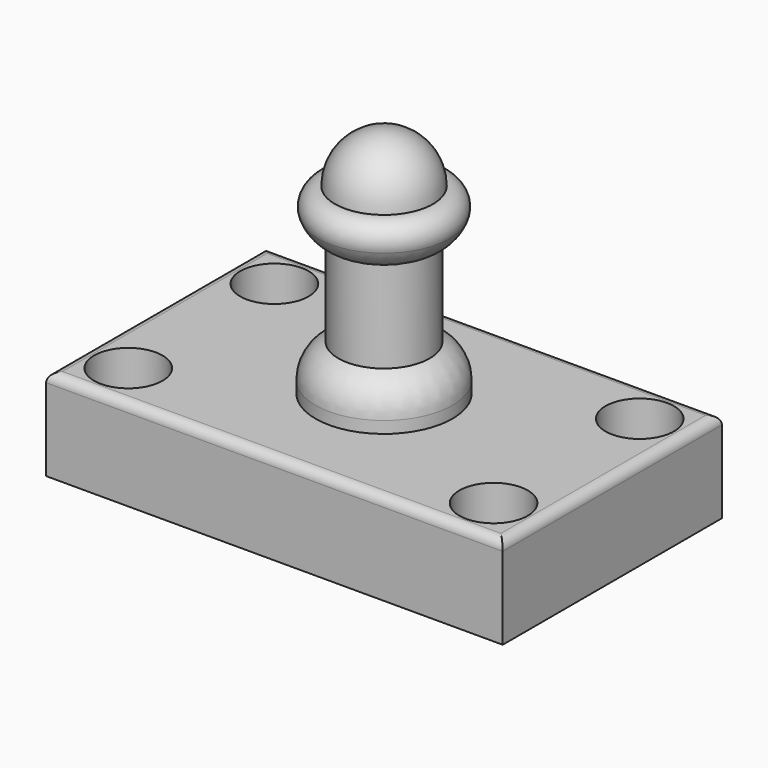
from build123d import *

# Parameters (mm, degrees)
F0_W     = 127
F0_H     = 76.2
F1_DEPTH = 25.4
F3_D     = 19.05
F4_W     = 19.05
F4_H     = 50.8
F6_W     = 12.7
F6_H     = 25.4
F9_R     = 2.54


# Not quite as in the source:
# - a fillet or chamfer that OpenCascade refuses, or shapes differently, is made with other operations: its cross-section is extruded or revolved along the edge and cut away or added


with BuildPart() as f1:
    # F0 (on Top) → F1 (new body)
    with BuildSketch(Plane.XY):
        Rectangle(F0_W, F0_H)
    extrude(amount=F1_DEPTH)

    # F3 (through all)
    with Locations(Plane.XY.offset(25.4)):
        with Locations((-50.8, 25.4), (50.8, 25.4), (-50.8, -25.4), (50.8, -25.4)):
            Hole(F3_D / 2)

    # F4 (on Front) → F5 (revolve)
    with BuildSketch(Plane.XZ):
        with Locations((-9.525, 50.8)):
            Rectangle(F4_W, F4_H)
    revolve(axis=Axis((0, 0, 50.8), (0, 0, 1)))

    # F6 (on Front) → F7 (revolve, cut)
    with BuildSketch(Plane.XZ):
        with Locations((-19.05, 50.8)):
            Rectangle(F6_W, F6_H)
    revolve(axis=Axis((0, 0, 50.8), (0, 0, -1)), mode=Mode.SUBTRACT)

    # F8: fillet of radius 10.16 on 2 edges, made by hand

    # F8_s1 → F8_t2 (revolve, cut)
    with BuildSketch(Plane.XZ):
        with BuildLine():
            ThreePointArc((-19.05, 28.6814279214), (-17.3142269675, 34.3610405842), (-12.7, 38.1))
            Line((-12.7, 38.1), (-19.05, 38.1))
            Line((-19.05, 38.1), (-19.05, 28.6814279214))
        make_face()
    revolve(axis=Axis((0, 0, 38.1), (0, 0, -1)), mode=Mode.SUBTRACT)

    # F8_s3 → F8_t4 (revolve, cut)
    with BuildSketch(Plane.XZ):
        with BuildLine():
            ThreePointArc((-12.7, 63.5), (-17.3142269675, 67.2389594158), (-19.05, 72.9185720786))
            Line((-19.05, 72.9185720786), (-19.05, 63.5))
            Line((-19.05, 63.5), (-12.7, 63.5))
        make_face()
    revolve(axis=Axis((0, 0, 63.5), (0, 0, -1)), mode=Mode.SUBTRACT)

    # F9
    f9_edges = [f1.edges().sort_by_distance(p)[0] for p in [
        (0, 38.1, 25.4),
        (63.5, 0, 25.4),
        (0, -38.1, 25.4),
        (-63.5, 0, 25.4),
    ]]
    fillet(f9_edges, radius=F9_R)

    # F10: fillet of radius 5.08 on 1 edges, made by hand

    # F10_s1 → F10_t2 (revolve, cut)
    with BuildSketch(Plane.XZ):
        with BuildLine():
            ThreePointArc((-18.3919026469, 69.3214279214), (-17.8208524084, 74.0070100312), (-13.6409513235, 76.2))
            Line((-13.6409513235, 76.2), (-13.6409513235, 76.708))
            Line((-13.6409513235, 76.708), (-19.05, 76.708))
            Line((-19.05, 76.708), (-19.558, 76.2))
            ThreePointArc((-19.558, 76.2), (-19.558, 72.9185720786), (-18.8669977793, 69.1415707135))
            Line((-18.8669977793, 69.1415707135), (-18.3919026469, 69.3214279214))
        make_face()
    revolve(axis=Axis((0, 0, 76.2), (0, 0, 1)), mode=Mode.SUBTRACT)

    # F11 (on Front) → F12 (revolve)
    with BuildSketch(Plane.XZ):
        with BuildLine():
            Line((0, 76.2), (0, 89.8398))
            ThreePointArc((0, 89.8398), (-9.710461042, 85.7786789481), (-13.638526776, 76.0136363248))
            Line((-13.638526776, 76.0136363248), (0, 76.2))
        make_face()
    revolve(axis=Axis((0, 0, 83.0199), (0, 0, -1)))


solid = f1.part
